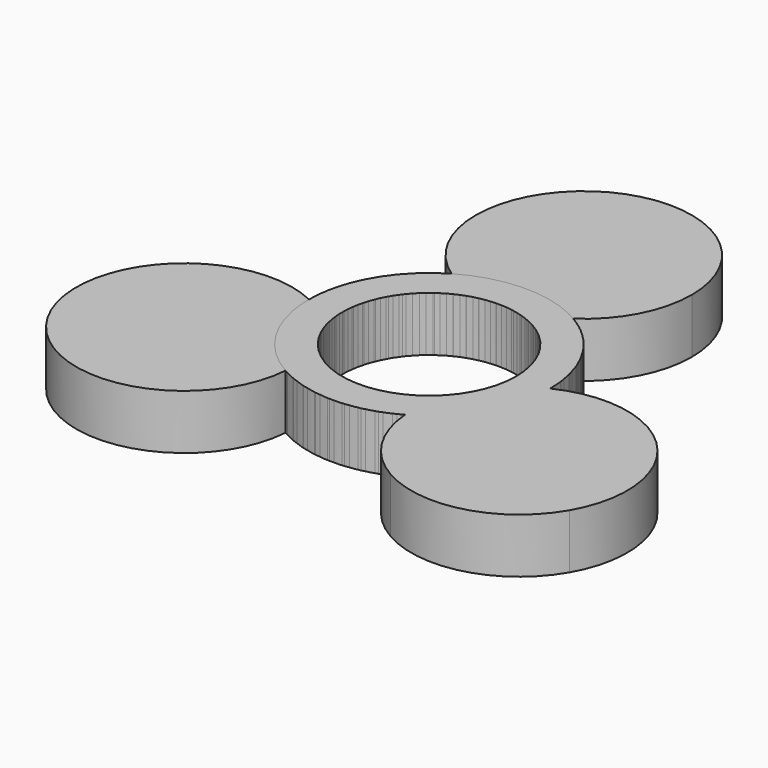
from build123d import *

# Parameters (mm, degrees)
F2_DEPTH        = 7
F2_COPIES_COUNT = 3


# Not quite as in the source:
# - a feature of the source that left no trace in its solid (it failed there, or was rolled back) is left out
# - a pattern or mirror of a feature is missing from the dataset's text; its kind, count and spacing are read off the source's solid
# - the program builds the solid bodies; features that only make, move or delete a surface that nothing else refers to are left out


with BuildPart() as f2:
    # F0 (on Top) → F2 (new body)
    with BuildSketch(Plane.XY):
        with BuildLine():
            ThreePointArc((0, 38.5565236211), (-13.2022888, 28.8154730257), (-7.7895226824, 13.3270754579))
            ThreePointArc((-7.7895226824, 13.3270754579), (-4.0350532405, 14.8998640674), (0, 15.4365671016))
            Line((0, 15.4365671016), (0, 38.5565236211))
        make_face()
        with BuildLine():
            ThreePointArc((0, 15.4365671016), (4.0350532405, 14.8998640674), (7.7895226824, 13.3270754579))
            ThreePointArc((7.7895226824, 13.3270754579), (12.2177156199, 18.2861624394), (13.8172209263, 24.7393026948))
            ThreePointArc((13.8172209263, 24.7393026948), (9.7702506141, 34.5095533089), (0, 38.5565236211))
            Line((0, 38.5565236211), (0, 15.4365671016))
        make_face()
        with BuildLine():
            ThreePointArc((-7.7895226824, 13.3270754579), (-4.8246777269, 11.7917902326), (-1.5781237611, 11.0124997342))
            ThreePointArc((-1.5781237611, 11.0124997342), (-0.7910643013, 11.0968392919), (0, 11.125))
            Line((0, 11.125), (0, 15.4365671016))
            ThreePointArc((0, 15.4365671016), (-4.0350532405, 14.8998640674), (-7.7895226824, 13.3270754579))
        make_face()
        with BuildLine():
            ThreePointArc((0, 11.125), (0.7910643013, 11.0968392919), (1.5781237611, 11.0124997342))
            ThreePointArc((1.5781237611, 11.0124997342), (4.8246777269, 11.7917902326), (7.7895226824, 13.3270754579))
            ThreePointArc((7.7895226824, 13.3270754579), (4.0350532405, 14.8998640674), (0, 15.4365671016))
            Line((0, 15.4365671016), (0, 11.125))
        make_face()
        with BuildLine():
            ThreePointArc((1.5781237611, 11.0124997342), (8.4060172449, 7.2872833813), (11.125, 0))
            ThreePointArc((11.125, 0), (-7.2872833813, -8.4060172449), (-1.5781237611, 11.0124997342))
            ThreePointArc((-1.5781237611, 11.0124997342), (-4.8246777269, 11.7917902326), (-7.7895226824, 13.3270754579))
            ThreePointArc((-7.7895226824, 13.3270754579), (-7.682581412, -13.3890084297), (15.4365671016, 0))
            ThreePointArc((15.4365671016, 0), (13.3890084297, 7.682581412), (7.7895226824, 13.3270754579))
            ThreePointArc((7.7895226824, 13.3270754579), (4.8246777269, 11.7917902326), (1.5781237611, 11.0124997342))
        make_face()
    extrude(amount=F2_DEPTH)


with BuildPart() as f2_copies_1:
    # F2_copies: instance of F2
    add(f2.part.rotate(Axis((0, 0, 0), (0, 0, 1)), 1 * 360 / F2_COPIES_COUNT))


with BuildPart() as f2_copies_2:
    # F2_copies: instance of F2
    add(f2.part.rotate(Axis((0, 0, 0), (0, 0, 1)), 2 * 360 / F2_COPIES_COUNT))


solid = Compound([f2.part, f2_copies_1.part, f2_copies_2.part])
